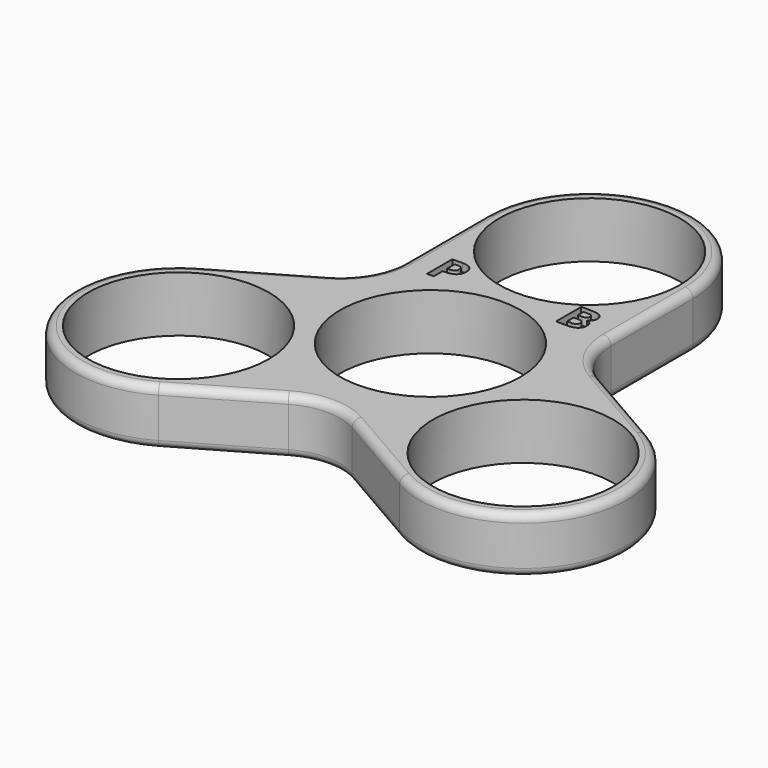
from build123d import *

# Parameters (mm, degrees)
F0_R         = 11.35
F1_DEPTH     = 7
F2_R         = 1
F3_TEXT_SIZE = 5.5555555556
F4_DEPTH     = 1


# Not quite as in the source:
# - Text() gives the source's letters only with a copy of the font that has no kerning and outlines rounded to 1/6400 em; it was checked with that copy


with BuildPart() as f1:
    # F0 (on Top) → F1 (new body)
    with BuildSketch(Plane.XY):
        with BuildLine():
            ThreePointArc((-13, 12.124355653), (-14.0717967697, 8.124355653), (-17, 5.1961524227))
            Line((-17, 5.1961524227), (-28.1506350946, -1.2416697508))
            ThreePointArc((-28.1506350946, -1.2416697508), (-32.9089653438, -19), (-15.1506350946, -23.7583302492))
            Line((-15.1506350946, -23.7583302492), (-4, -17.3205080757))
            ThreePointArc((-4, -17.3205080757), (0, -16.248711306), (4, -17.3205080757))
            Line((4, -17.3205080757), (15.1506350946, -23.7583302492))
            ThreePointArc((15.1506350946, -23.7583302492), (32.9089653438, -19), (28.1506350946, -1.2416697508))
            Line((28.1506350946, -1.2416697508), (17, 5.1961524227))
            ThreePointArc((17, 5.1961524227), (14.0717967697, 8.124355653), (13, 12.124355653))
            Line((13, 12.124355653), (13, 25))
            ThreePointArc((13, 25), (0, 38), (-13, 25))
            Line((-13, 25), (-13, 12.124355653))
        make_face()
        with Locations((-21.6506350946, -12.5)):
            Circle(F0_R, mode=Mode.SUBTRACT)
        Circle(F0_R, mode=Mode.SUBTRACT)
        with Locations((21.6506350946, -12.5)):
            Circle(F0_R, mode=Mode.SUBTRACT)
        with Locations((0, 25)):
            Circle(F0_R, mode=Mode.SUBTRACT)
    extrude(amount=F1_DEPTH)

    # F2
    f2_edges = [f1.edges().sort_by_distance(p)[0] for p in [
        (-14.071797, 8.124356, 7),
        (-14.071797, 8.124356, 0),
    ]]
    fillet(f2_edges, radius=F2_R)

    # F3 (on face) → F4 (cut)
    with BuildSketch(Plane.XY.offset(7)):
        with Locations((-10, 11.35)):
            Text('P', F3_TEXT_SIZE, font='Open Sans', font_style=FontStyle.BOLD, text_align=(TextAlign.LEFT, TextAlign.BOTTOM))
        with Locations((6.1996527778, 11.35)):
            Text('B', F3_TEXT_SIZE, font='Open Sans', font_style=FontStyle.BOLD, text_align=(TextAlign.LEFT, TextAlign.BOTTOM))
    extrude(amount=-F4_DEPTH, mode=Mode.SUBTRACT)


solid = f1.part
